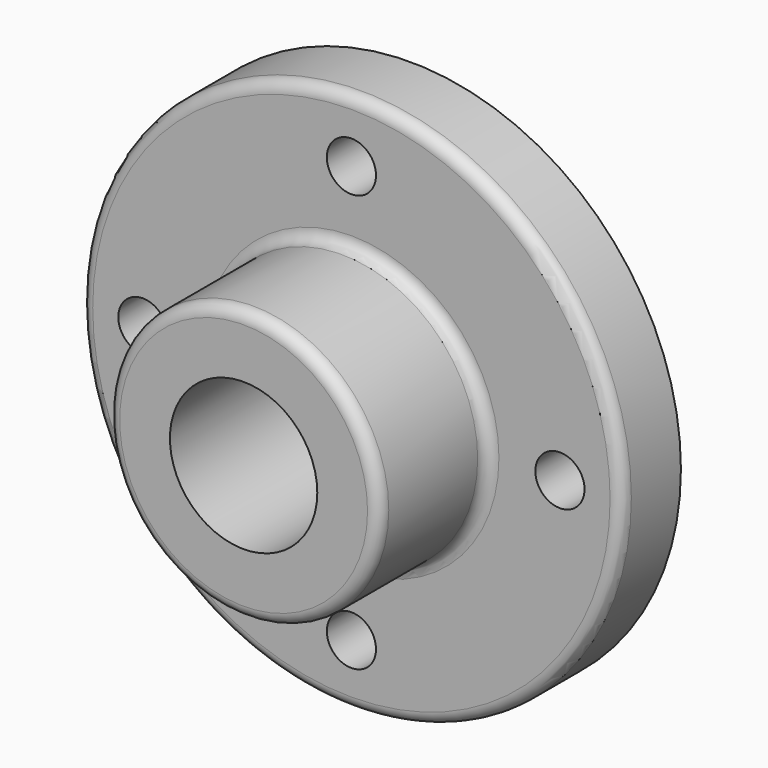
from build123d import *

# Parameters (mm, degrees)
F0_R            = 69.85
F1_DEPTH        = 19.05
F2_R            = 35.052
F3_DEPTH        = 34.798
F4_R            = 19.0246
F5_DEPTH        = 53.849
F6_R            = 6.35
F7_DEPTH        = 19.051
F7_COPIES_COUNT = 4
F8_R            = 3.048


# Not quite as in the source:
# - a pattern or mirror of a feature is missing from the dataset's text; its kind, count and spacing are read off the source's solid


with BuildPart() as f1:
    # F0 (on Front) → F1 (new body)
    with BuildSketch(Plane.XZ):
        Circle(F0_R)
    extrude(amount=-F1_DEPTH)

    # F2 (on face) → F3 (join)
    with BuildSketch(Plane.XZ):
        Circle(F2_R)
    extrude(amount=F3_DEPTH)

    # F4 (on face) → F5 (cut, through all)
    with BuildSketch(Plane.XZ.offset(34.798)):
        Circle(F4_R)
    extrude(amount=-F5_DEPTH, mode=Mode.SUBTRACT)

    # F6 (on face) → F7 (cut, through all)
    with BuildSketch(Plane.XZ):
        with Locations((0, 53.848)):
            Circle(F6_R)
    f7 = extrude(amount=-F7_DEPTH, mode=Mode.SUBTRACT)

    # F7_copies: F7 ×4 about axis
    f7_copies_axis = Axis((0, 0, 0), (0, 1, 0))
    for i in range(1, F7_COPIES_COUNT):
        add(f7.rotate(f7_copies_axis, i * 360 / F7_COPIES_COUNT), mode=Mode.SUBTRACT)

    # F8
    f8_edges = [f1.edges().sort_by_distance(p)[0] for p in [
        (-35.052, -34.798, 0),
        (-35.052, 0, 0),
        (-69.85, 0, 0),
    ]]
    fillet(f8_edges, radius=F8_R)


solid = f1.part
